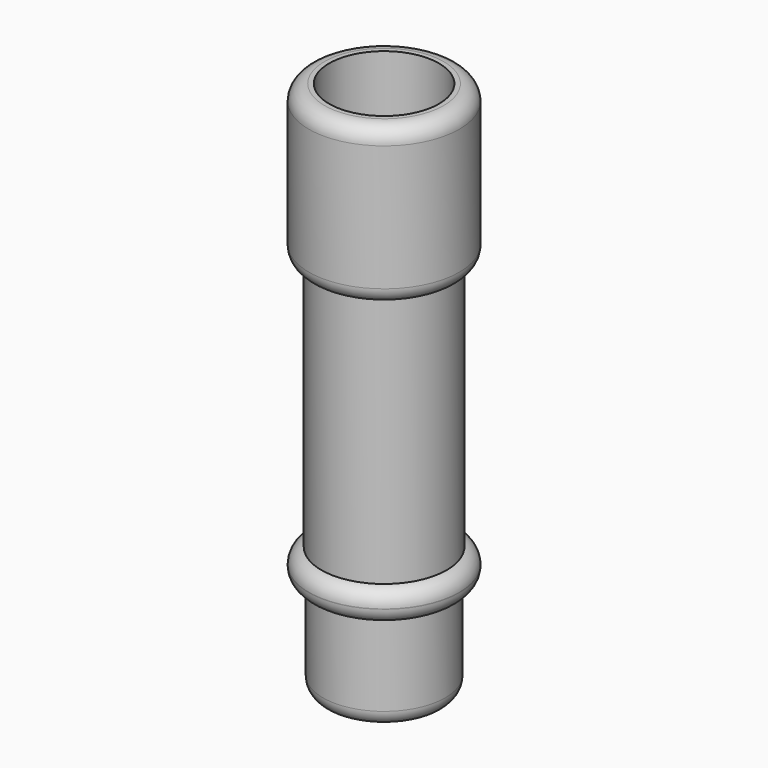
from build123d import *

# Parameters (mm, degrees)
F0_R     = 19.5
F0_R_2   = 17.5
F1_DEPTH = 30
F2_R     = 24
F2_R_2   = 19.5
F2_R_3   = 17.5
F3_DEPTH = 10
F4_R     = 20
F4_R_2   = 17.5
F5_DEPTH = 80
F6_R     = 24
F6_R_2   = 17.5
F7_DEPTH = 50


# Not quite as in the source:
# - a fillet or chamfer that OpenCascade refuses, or shapes differently, is made with other operations: its cross-section is extruded or revolved along the edge and cut away or added


with BuildPart() as f1:
    # F0 (on Top) → F1 (new body)
    with BuildSketch(Plane.XY):
        Circle(F0_R)
        Circle(F0_R_2, mode=Mode.SUBTRACT)
    extrude(amount=F1_DEPTH)

    # F2 (on face) → F3 (join)
    with BuildSketch(Plane.XY.offset(30)):
        Circle(F2_R)
        Circle(F2_R_2, mode=Mode.SUBTRACT)
        Circle(F2_R_2)
        Circle(F2_R_3, mode=Mode.SUBTRACT)
    extrude(amount=F3_DEPTH)

    # F4 (on face) → F5 (join)
    with BuildSketch(Plane.XY.offset(40)):
        Circle(F4_R)
        Circle(F4_R_2, mode=Mode.SUBTRACT)
    extrude(amount=F5_DEPTH)

    # F6 (on face) → F7 (join)
    with BuildSketch(Plane.XY.offset(120)):
        Circle(F6_R)
        Circle(F6_R_2, mode=Mode.SUBTRACT)
    extrude(amount=F7_DEPTH)

    # F8: fillet of radius 5 on 5 edges, made by hand

    # F8_s1 → F8_t2 (revolve, cut)
    with BuildSketch(Plane.XZ):
        with BuildLine():
            ThreePointArc((24, 165), (22.5355339059, 168.5355339059), (19, 170))
            Line((19, 170), (24, 170))
            Line((24, 170), (24, 165))
        make_face()
    revolve(axis=Axis((0, 0, 170), (0, 0, 1)), mode=Mode.SUBTRACT)

    # F8_s3 → F8_t4 (revolve, cut)
    with BuildSketch(Plane.XZ):
        with BuildLine():
            ThreePointArc((20, 120), (22.8729833462, 121.7367018254), (24, 124.8989794856))
            Line((24, 124.8989794856), (24, 120))
            Line((24, 120), (20, 120))
        make_face()
    revolve(axis=Axis((0, 0, 120), (0, 0, 1)), mode=Mode.SUBTRACT)

    # F8_s5 → F8_t6 (revolve, cut)
    with BuildSketch(Plane.XZ):
        with BuildLine():
            ThreePointArc((24, 35.1010205144), (22.8729833462, 38.2632981746), (20, 40))
            Line((20, 40), (24, 40))
            Line((24, 40), (24, 35.1010205144))
        make_face()
    revolve(axis=Axis((0, 0, 40), (0, 0, 1)), mode=Mode.SUBTRACT)

    # F8_s7 → F8_t8 (revolve, cut)
    with BuildSketch(Plane.XZ):
        with BuildLine():
            ThreePointArc((19.5, 30), (22.7080992435, 31.6208352193), (24, 34.9749371855))
            Line((24, 34.9749371855), (24, 30))
            Line((24, 30), (19.5, 30))
        make_face()
    revolve(axis=Axis((0, 0, 30), (0, 0, 1)), mode=Mode.SUBTRACT)

    # F8_s9 → F8_t10 (revolve, cut)
    with BuildSketch(Plane.XZ):
        with BuildLine():
            ThreePointArc((19.5, 4), (18.972135955, 1.7639320225), (17.5, 0))
            Line((17.5, 0), (19.5, 0))
            Line((19.5, 0), (19.5, 4))
        make_face()
    revolve(axis=Axis((0, 0, 0), (0, 0, 1)), mode=Mode.SUBTRACT)


solid = f1.part
